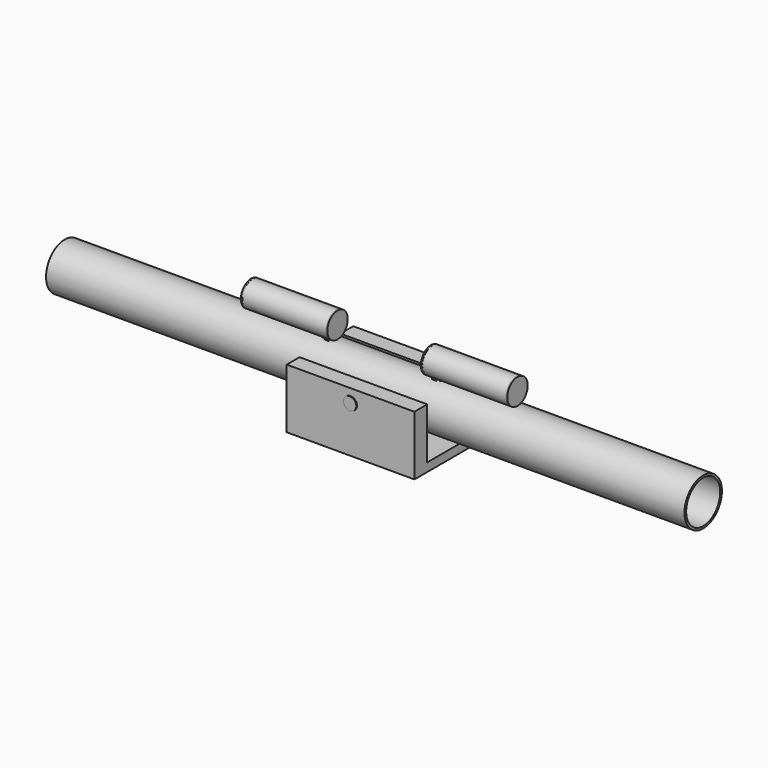
from build123d import *

# Parameters (mm, degrees)
F0_R          = 55
F0_R_2        = 50
F1_DEPTH      = 1500
F4_DEPTH      = 300
F6_R          = 15
F7_DEPTH      = 100
F7_DEPTH_BACK = 100
F8_R          = 30
F8_R_2        = 25
F9_DEPTH      = 200
F13_R         = 30
F14_DEPTH     = 3
F17_DEPTH     = 25
F23_W         = 15
F23_H         = 15
F24_DEPTH     = 10
F29_R         = 7.5
F30_DEPTH     = 10


# Not quite as in the source:
# - a feature names something its author has since deleted; it is built from what else it names


with BuildPart() as f1:
    # F0 (on Right) → F1 (new body)
    with BuildSketch(Plane.YZ):
        Circle(F0_R)
        Circle(F0_R_2, mode=Mode.SUBTRACT)
    extrude(amount=F1_DEPTH)


with BuildPart() as f1_1:
    # F2: moved
    add(f1.part.moved(Location((-750, 0, 0))))


with BuildPart() as f4:
    # F3 (on Right) → F4 (new body)
    with BuildSketch(Plane.YZ):
        Polygon((317.1720561673, -27.7593303259), (279.5250168443, -27.7593303259), (279.5250168443, -147.7593303259), (159.5250168443, -147.7593303259), (159.5250168443, -27.7593303259), (121.8779775212, -27.7593303259), (121.8779775212, -167.7593303259), (317.1720561673, -167.7593303259), align=None)
    extrude(amount=F4_DEPTH)


with BuildPart() as f4_1:
    # F5: moved
    add(f4.part.moved(Location((-150, -220, 59))))


with BuildPart() as f7:
    # F6 (on Front) → F7 (new body, two sides)
    with BuildSketch(Plane.XZ) as f7_sk:
        Circle(F6_R)
    extrude(amount=F7_DEPTH)
    extrude(f7_sk.sketch, amount=-F7_DEPTH_BACK)


with BuildPart() as f9:
    # F8 (on Right) → F9 (new body)
    with BuildSketch(Plane.YZ):
        with Locations((8.1081893295, 102.8191223741)):
            Circle(F8_R)
        with Locations((8.1081893295, 102.8191223741)):
            Circle(F8_R_2, mode=Mode.SUBTRACT)
    extrude(amount=F9_DEPTH)


with BuildPart() as f9_1:
    # F10: moved
    add(f9.part.moved(Location((-421, -7, 60))))


with BuildPart() as f14:
    # F13 (on offset) → F14 (new body)
    with BuildSketch(Plane(origin=(-446, 0, 0), x_dir=(0, -1, 0), z_dir=(-1, 0, 0))):
        with Locations((0, 176.3660857303)):
            Circle(F13_R)
    extrude(amount=F14_DEPTH)


with BuildPart() as f14_1:
    # F15: moved
    add(f14.part.moved(Location((26.1, 0.9, -13.4))))


with BuildPart() as f16_1:
    # F16: copy of F14
    add(f14_1.part.moved(Location((200, 0, 0))))


with BuildPart() as f17:
    # F11 (on Front) → F17 (new body)
    with BuildSketch(Plane.XZ):
        Polygon((-9.3342950797, 103.075656802), (-19.3342950797, 103.075656802), (-19.3342950797, 83.075656802), (-39.3342950797, 83.075656802), (-39.3342950797, 73.075656802), (-9.3342950797, 73.075656802), align=None)
    extrude(amount=F17_DEPTH)


with BuildPart() as f18_1:
    # F18: copy of F17
    add(f17.part.moved(Location((0, 0, 60))))


with BuildPart() as f18_1_1:
    # F19: moved
    add(f18_1.part.moved(Location((-225, 14, -21.2))))


with BuildPart() as f9_2:
    # F20: moved
    add(f9_1.part.moved(Location((110, 0, 0))))


with BuildPart() as f16_1_1:
    # F20: moved
    add(f16_1.part.moved(Location((110, 0, 0))))


with BuildPart() as f18_1_2:
    # F20: moved
    add(f18_1_1.part.moved(Location((110, 0, 0))))


with BuildPart() as f14_2:
    # F20: moved
    add(f14_1.part.moved(Location((110, 0, 0))))


with BuildPart() as f18_1_3:
    # F22: moved
    add(f18_1_2.part.moved(Location((232, 0, 67))))


with BuildPart() as f24:
    # F23 (on Top) → F24 (new body)
    with BuildSketch(Plane.XY):
        with Locations((-226.4265790582, 107.5248345733)):
            Rectangle(F23_W, F23_H)
    extrude(amount=F24_DEPTH)


with BuildPart() as f24_1:
    # F25: moved
    add(f24.part.moved(Location((89, -106.8, 129))))


with BuildPart() as f9_3:
    add(f9_2.part)

    # F26: cut F24
    add(f24_1.part, mode=Mode.SUBTRACT)


with BuildPart() as f18_1_4:
    # F27: moved
    add(f18_1_3.part.moved(Location((-229.1, 0, -66))))


with BuildPart() as f28_1:
    # F28: instance of F9
    add(f9_3.part.mirror(Plane.YZ))


with BuildPart() as f28_2:
    # F28: instance of F16_1
    add(f16_1_1.part.mirror(Plane.YZ))


with BuildPart() as f28_3:
    # F28: instance of F18_1
    add(f18_1_4.part.mirror(Plane.YZ))


with BuildPart() as f28_4:
    # F28: instance of F14
    add(f14_2.part.mirror(Plane.YZ))


with BuildPart() as f30:
    # F29 (on Top) → F30 (new body)
    with BuildSketch(Plane.XY):
        with Locations((-268.535554409, 105.6018322706)):
            Circle(F29_R)
    extrude(amount=F30_DEPTH)


with BuildPart() as f30_1:
    # F31: moved
    add(f30.part.moved(Location((131, -106, 48))))


with BuildPart() as f32_1:
    # F32: copy of F30
    add(f30_1.part.moved(Location((275, 0, 0))))


with BuildPart() as f1_2:
    add(f1_1.part)

    # F33: cut F30, F32_1
    add(f30_1.part, mode=Mode.SUBTRACT)
    add(f32_1.part, mode=Mode.SUBTRACT)


with BuildPart() as f9_4:
    # F34: moved
    add(f9_3.part.moved(Location((0, 0, -77))))


with BuildPart() as f16_1_2:
    # F34: moved
    add(f16_1_1.part.moved(Location((0, 0, -77))))


with BuildPart() as f28_1_1:
    # F34: moved
    add(f28_1.part.moved(Location((0, 0, -77))))


with BuildPart() as f18_1_5:
    # F34: moved
    add(f18_1_4.part.moved(Location((0, 0, -77))))


with BuildPart() as f14_3:
    # F34: moved
    add(f14_2.part.moved(Location((0, 0, -77))))


with BuildPart() as f28_4_1:
    # F34: moved
    add(f28_4.part.moved(Location((0, 0, -77))))


with BuildPart() as f28_2_1:
    # F34: moved
    add(f28_2.part.moved(Location((0, 0, -77))))


with BuildPart() as f28_3_1:
    # F34: moved
    add(f28_3.part.moved(Location((0, 0, -77))))


solid = Compound([f4_1.part, f7.part, f1_2.part, f9_4.part, f16_1_2.part, f28_1_1.part, f18_1_5.part, f14_3.part, f28_4_1.part, f28_2_1.part, f28_3_1.part])
